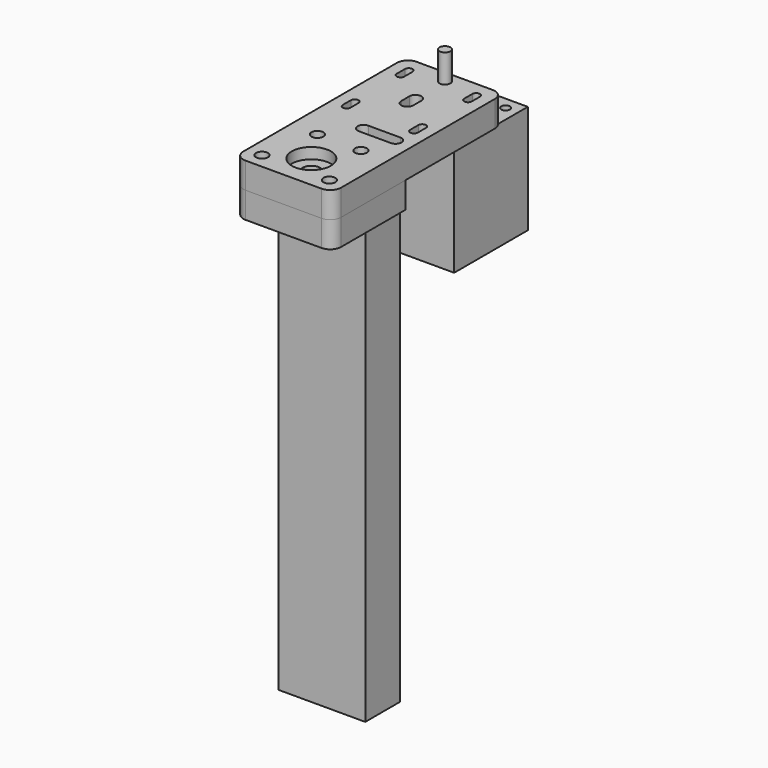
from build123d import *

# Parameters (mm, degrees)
F1_R      = 11
F1_R_2    = 4
F2_DEPTH  = 7
F0_W      = 42.3
F0_H      = 42.3
F0_R      = 2
F0_R_2    = 11
F0_R_3    = 2.5
F3_DEPTH  = 50
F4_DEPTH  = 2
F5_DEPTH  = 25
F6_R      = 2.75
F6_R_2    = 11
F6_R_3    = 9
F7_DEPTH  = 12
F8_DEPTH  = 7
F9_DEPTH  = 3
F10_DEPTH = 12
F11_DEPTH = 7
F12_W     = 40
F12_H     = 20
F12_R     = 2.5
F13_DEPTH = 200
F14_DEPTH = 4.5


with BuildPart() as f2:
    # F1 (on Top) → F2 (new body)
    with BuildSketch(Plane.XY):
        Circle(F1_R)
        Circle(F1_R_2, mode=Mode.SUBTRACT)
    extrude(amount=F2_DEPTH)


with BuildPart() as f3:
    # F0 (on Top) → F3 (new body)
    with BuildSketch(Plane.XY):
        with Locations((0, 76.8215209246)):
            Rectangle(F0_W, F0_H)
        with Locations((-15.5, 61.3215209246)):
            Circle(F0_R, mode=Mode.SUBTRACT)
        with Locations((15.5, 61.3215209246)):
            Circle(F0_R, mode=Mode.SUBTRACT)
        with Locations((-15.5, 92.3215209246)):
            Circle(F0_R, mode=Mode.SUBTRACT)
        with Locations((0, 76.8215209246)):
            Circle(F0_R_2, mode=Mode.SUBTRACT)
        with Locations((15.5, 92.3215209246)):
            Circle(F0_R, mode=Mode.SUBTRACT)
        with Locations((0, 76.8215209246)):
            Circle(F0_R_2)
        with Locations((0, 76.8215209246)):
            Circle(F0_R_3, mode=Mode.SUBTRACT)
    extrude(amount=-F3_DEPTH)

    # F0 (on Top) → F4 (join)
    with BuildSketch(Plane.XY):
        with Locations((0, 76.8215209246)):
            Circle(F0_R_2)
        with Locations((0, 76.8215209246)):
            Circle(F0_R_3, mode=Mode.SUBTRACT)
    extrude(amount=F4_DEPTH)

    # F0 (on Top) → F5 (join)
    with BuildSketch(Plane.XY):
        with Locations((0, 76.8215209246)):
            Circle(F0_R_3)
    extrude(amount=F5_DEPTH)


with BuildPart() as f7:
    # F6 (on Top) → F7 (new body)
    with BuildSketch(Plane.XY):
        with BuildLine():
            Line((17.0594010768, 26), (22.5, 26))
            Line((22.5, 26), (22.5, 77.35))
            ThreePointArc((22.5, 77.35), (21.0355339059, 80.8855339059), (17.5, 82.35))
            Line((17.5, 82.35), (-17.5, 82.35))
            ThreePointArc((-17.5, 82.35), (-21.0355339059, 80.8855339059), (-22.5, 77.35))
            Line((-22.5, 77.35), (-22.5, 26))
            Line((-22.5, 26), (-2.3094010768, 26))
            Line((-2.3094010768, 26), (-4.6188021535, 30))
            Line((-4.6188021535, 30), (-2.3094010768, 34))
            Line((-2.3094010768, 34), (17.0594010768, 34))
            Line((17.0594010768, 34), (19.3688021535, 30))
            Line((19.3688021535, 30), (17.0594010768, 26))
        make_face()
        with BuildLine():
            Line((-17.25, 39.65), (-17.25, 44.35))
            ThreePointArc((-17.25, 44.35), (-15.5, 46.1), (-13.75, 44.35))
            Line((-13.75, 44.35), (-13.75, 39.65))
            ThreePointArc((-13.75, 39.65), (-15.5, 37.9), (-17.25, 39.65))
        make_face(mode=Mode.SUBTRACT)
        with BuildLine():
            Line((-17.25, 70.65), (-17.25, 75.35))
            ThreePointArc((-17.25, 75.35), (-15.5, 77.1), (-13.75, 75.35))
            Line((-13.75, 75.35), (-13.75, 70.65))
            ThreePointArc((-13.75, 70.65), (-15.5, 68.9), (-17.25, 70.65))
        make_face(mode=Mode.SUBTRACT)
        with BuildLine():
            ThreePointArc((11.5, 55.15), (0, 43.65), (-11.5, 55.15))
            Line((-11.5, 55.15), (-11.5, 59.85))
            ThreePointArc((-11.5, 59.85), (0, 71.35), (11.5, 59.85))
            Line((11.5, 59.85), (11.5, 55.15))
        make_face(mode=Mode.SUBTRACT)
        with BuildLine():
            Line((13.75, 39.65), (13.75, 44.35))
            ThreePointArc((13.75, 44.35), (15.5, 46.1), (17.25, 44.35))
            Line((17.25, 44.35), (17.25, 39.65))
            ThreePointArc((17.25, 39.65), (15.5, 37.9), (13.75, 39.65))
        make_face(mode=Mode.SUBTRACT)
        with BuildLine():
            Line((13.75, 70.65), (13.75, 75.35))
            ThreePointArc((13.75, 75.35), (15.5, 77.1), (17.25, 75.35))
            Line((17.25, 75.35), (17.25, 70.65))
            ThreePointArc((17.25, 70.65), (15.5, 68.9), (13.75, 70.65))
        make_face(mode=Mode.SUBTRACT)
        with BuildLine():
            Line((-17.5, -16), (0, -16))
            Line((0, -16), (17.5, -16))
            ThreePointArc((17.5, -16), (21.0355339059, -14.5355339059), (22.5, -11))
            Line((22.5, -11), (22.5, 26))
            Line((22.5, 26), (17.0594010768, 26))
            Line((17.0594010768, 26), (-2.3094010768, 26))
            Line((-2.3094010768, 26), (-22.5, 26))
            Line((-22.5, 26), (-22.5, -11))
            ThreePointArc((-22.5, -11), (-21.0355339059, -14.5355339059), (-17.5, -16))
        make_face()
        with Locations((-15.5, -9)):
            Circle(F6_R, mode=Mode.SUBTRACT)
        with Locations((-10, 16)):
            Circle(F6_R, mode=Mode.SUBTRACT)
        Circle(F6_R_2, mode=Mode.SUBTRACT)
        with Locations((15.5, -9)):
            Circle(F6_R, mode=Mode.SUBTRACT)
        with Locations((10, 16)):
            Circle(F6_R, mode=Mode.SUBTRACT)
        with BuildLine():
            Line((-11.5, 59.85), (-11.5, 55.15))
            ThreePointArc((-11.5, 55.15), (0, 43.65), (11.5, 55.15))
            Line((11.5, 55.15), (11.5, 59.85))
            ThreePointArc((11.5, 59.85), (0, 71.35), (-11.5, 59.85))
        make_face()
        with BuildLine():
            Line((-2.75, 55.15), (-2.75, 59.85))
            ThreePointArc((-2.75, 59.85), (0, 62.6), (2.75, 59.85))
            Line((2.75, 59.85), (2.75, 55.15))
            ThreePointArc((2.75, 55.15), (0, 52.4), (-2.75, 55.15))
        make_face(mode=Mode.SUBTRACT)
        Circle(F6_R_2)
        Circle(F6_R_3, mode=Mode.SUBTRACT)
        Polygon((-2.3094010768, 26), (17.0594010768, 26), (19.3688021535, 30), (17.0594010768, 34), (-2.3094010768, 34), (-4.6188021535, 30), align=None)
        with BuildLine():
            Line((14.75, 27.25), (0, 27.25))
            ThreePointArc((0, 27.25), (-2.75, 30), (0, 32.75))
            Line((0, 32.75), (14.75, 32.75))
            ThreePointArc((14.75, 32.75), (17.5, 30), (14.75, 27.25))
        make_face(mode=Mode.SUBTRACT)
    extrude(amount=F7_DEPTH)

    # F6 (on Top) → F8 (cut)
    with BuildSketch(Plane.XY):
        Circle(F6_R_2)
        Circle(F6_R_3, mode=Mode.SUBTRACT)
    extrude(amount=F8_DEPTH, mode=Mode.SUBTRACT)

    # F6 (on Top) → F9 (cut)
    with BuildSketch(Plane.XY):
        with BuildLine():
            Line((-11.5, 59.85), (-11.5, 55.15))
            ThreePointArc((-11.5, 55.15), (0, 43.65), (11.5, 55.15))
            Line((11.5, 55.15), (11.5, 59.85))
            ThreePointArc((11.5, 59.85), (0, 71.35), (-11.5, 59.85))
        make_face()
        with BuildLine():
            Line((-2.75, 55.15), (-2.75, 59.85))
            ThreePointArc((-2.75, 59.85), (0, 62.6), (2.75, 59.85))
            Line((2.75, 59.85), (2.75, 55.15))
            ThreePointArc((2.75, 55.15), (0, 52.4), (-2.75, 55.15))
        make_face(mode=Mode.SUBTRACT)
    extrude(amount=F9_DEPTH, mode=Mode.SUBTRACT)

    # F6 (on Top) → F14 (cut)
    with BuildSketch(Plane.XY):
        Polygon((-2.3094010768, 26), (17.0594010768, 26), (19.3688021535, 30), (17.0594010768, 34), (-2.3094010768, 34), (-4.6188021535, 30), align=None)
        with BuildLine():
            Line((14.75, 27.25), (0, 27.25))
            ThreePointArc((0, 27.25), (-2.75, 30), (0, 32.75))
            Line((0, 32.75), (14.75, 32.75))
            ThreePointArc((14.75, 32.75), (17.5, 30), (14.75, 27.25))
        make_face(mode=Mode.SUBTRACT)
    extrude(amount=F14_DEPTH, mode=Mode.SUBTRACT)


with BuildPart() as f10:
    # F6 (on Top) → F10 (new body)
    with BuildSketch(Plane.XY):
        with BuildLine():
            Line((-17.5, -16), (0, -16))
            Line((0, -16), (17.5, -16))
            ThreePointArc((17.5, -16), (21.0355339059, -14.5355339059), (22.5, -11))
            Line((22.5, -11), (22.5, 26))
            Line((22.5, 26), (17.0594010768, 26))
            Line((17.0594010768, 26), (-2.3094010768, 26))
            Line((-2.3094010768, 26), (-22.5, 26))
            Line((-22.5, 26), (-22.5, -11))
            ThreePointArc((-22.5, -11), (-21.0355339059, -14.5355339059), (-17.5, -16))
        make_face()
        with Locations((-15.5, -9)):
            Circle(F6_R, mode=Mode.SUBTRACT)
        with Locations((-10, 16)):
            Circle(F6_R, mode=Mode.SUBTRACT)
        Circle(F6_R_2, mode=Mode.SUBTRACT)
        with Locations((15.5, -9)):
            Circle(F6_R, mode=Mode.SUBTRACT)
        with Locations((10, 16)):
            Circle(F6_R, mode=Mode.SUBTRACT)
        Circle(F6_R_2)
        Circle(F6_R_3, mode=Mode.SUBTRACT)
    extrude(amount=-F10_DEPTH)

    # F6 (on Top) → F11 (cut)
    with BuildSketch(Plane.XY):
        Circle(F6_R_2)
        Circle(F6_R_3, mode=Mode.SUBTRACT)
    extrude(amount=-F11_DEPTH, mode=Mode.SUBTRACT)


with BuildPart() as f13:
    # F12 (on face) → F13 (new body)
    with BuildSketch(Plane(origin=(0, 0, -12), x_dir=(1, 0, 0), z_dir=(0, 0, -1))):
        with Locations((0, -16)):
            Rectangle(F12_W, F12_H)
        with Locations((-10, -16)):
            Circle(F12_R, mode=Mode.SUBTRACT)
        with Locations((10, -16)):
            Circle(F12_R, mode=Mode.SUBTRACT)
    extrude(amount=F13_DEPTH)


solid = Compound([f2.part, f3.part, f7.part, f10.part, f13.part])
